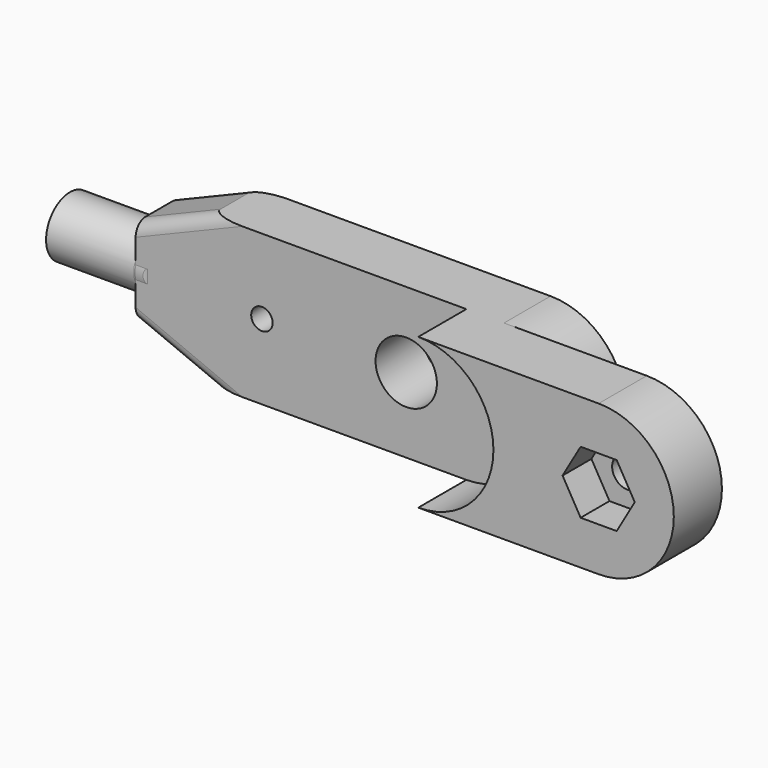
from build123d import *

# Parameters (mm, degrees)
F0_W         = 69.85
F0_H         = 15.875
F1_DEPTH     = 6.1468
F2_R         = 3.2385
F2_R_2       = 1.1303
F3_DEPTH     = 6.1478
F4_R         = 3.1496
F4_R_2       = 1.7272
F5_DEPTH     = 9.398
F7_T4_DEPTH  = 7.7320616198
F7_S5_R      = 3.1496
F7_T6_DEPTH  = 5
F7_T10_DEPTH = 7.7320616198
F7_S11_R     = 3.1496
F7_T12_DEPTH = 5
F9_DEPTH     = 25.4
F11_DEPTH    = 25.4
F13_DEPTH    = 6.35
F14_R        = 1.6256
F15_DEPTH    = 25.4
F17_DEPTH    = 3.81
F18_R        = 1.27


# Not quite as in the source:
# - a fillet or chamfer that OpenCascade refuses, or shapes differently, is made with other operations: its cross-section is extruded or revolved along the edge and cut away or added


with BuildPart() as f1:
    # F0 (on Front) → F1 (new body)
    with BuildSketch(Plane.XZ):
        Rectangle(F0_W, F0_H)
    extrude(amount=F1_DEPTH)

    # F2 (on face) → F3 (cut, through all)
    with BuildSketch(Plane.XZ.offset(6.1468)):
        with Locations((-6.35, 0)):
            Circle(F2_R)
        with Locations((-21.59, 0)):
            Circle(F2_R_2)
    extrude(amount=-F3_DEPTH, mode=Mode.SUBTRACT)

    # F4 (on face) → F5 (join)
    with BuildSketch(Plane(origin=(-34.925, 0, 0), x_dir=(0, -1, 0), z_dir=(-1, 0, 0))):
        with Locations((3.0734, 0)):
            Circle(F4_R)
        with Locations((3.0734, 0)):
            Circle(F4_R_2, mode=Mode.SUBTRACT)
    extrude(amount=F5_DEPTH)

    # F7: fillet of radius 1.27 on 6 edges, made by hand


with BuildPart() as f7_tool2:
    # F7_s3 → F7_t4 (new body)
    with BuildSketch(Plane.XY.offset(3.8660308099)):
        with BuildLine():
            ThreePointArc((-33.6540343146, -0.0004), (-34.5530256121, 0.3719743879), (-34.9254, 1.2709656854))
            Line((-34.9254, 1.2709656854), (-35.0525365685, 1.2709656854))
            ThreePointArc((-35.0525365685, 1.2709656854), (-35.0521365685, 0.6354828427), (-35.0521365685, 0))
            Line((-35.0521365685, 0), (-34.925, -0.1271365685))
            ThreePointArc((-34.925, -0.1271365685), (-34.2895171573, -0.1271365685), (-33.6540343146, -0.1275365685))
            Line((-33.6540343146, -0.1275365685), (-33.6540343146, -0.0004))
        make_face()
    extrude(amount=-F7_T4_DEPTH)

    # F7_s5 → F7_t6 (intersect, symmetric)
    with BuildSketch(Plane.YZ.offset(-34.4)):
        with Locations((-3.0734, 0)):
            Circle(F7_S5_R)
    extrude(amount=F7_T6_DEPTH, both=True, mode=Mode.INTERSECT)


with BuildPart() as f1_1:
    add(f1.part)

    # F7_t1: union F7_tool2
    add(f7_tool2.part)


with BuildPart() as f7_tool8:
    # F7_s9 → F7_t10 (new body)
    with BuildSketch(Plane.XY.offset(3.8660308099)):
        with BuildLine():
            ThreePointArc((-33.6540343146, -6.1464), (-34.5530256121, -6.5187743879), (-34.9254, -7.4177656854))
            Line((-34.9254, -7.4177656854), (-35.0525365685, -7.4177656854))
            ThreePointArc((-35.0525365685, -7.4177656854), (-35.0521365685, -6.7822828427), (-35.0521365685, -6.1468))
            Line((-35.0521365685, -6.1468), (-34.925, -6.0196634315))
            ThreePointArc((-34.925, -6.0196634315), (-34.2895171573, -6.0196634315), (-33.6540343146, -6.0192634315))
            Line((-33.6540343146, -6.0192634315), (-33.6540343146, -6.1464))
        make_face()
    extrude(amount=-F7_T10_DEPTH)

    # F7_s11 → F7_t12 (intersect, symmetric)
    with BuildSketch(Plane.YZ.offset(-34.4)):
        with Locations((-3.0734, 0)):
            Circle(F7_S11_R)
    extrude(amount=F7_T12_DEPTH, both=True, mode=Mode.INTERSECT)


with BuildPart() as f1_2:
    add(f1_1.part)

    # F7_t7: union F7_tool8
    add(f7_tool8.part)

    # F8 (on face) → F9 (cut)
    with BuildSketch(Plane.XZ.offset(6.1468)):
        Polygon((-34.925, 4.6355), (-26.9748, 7.9375), (-34.925, 7.9375), align=None)
        Polygon((-34.925, -7.9375), (-26.9748, -7.9375), (-34.925, -4.6355), align=None)
    extrude(amount=-F9_DEPTH, mode=Mode.SUBTRACT)

    # F10 (on face) → F11 (cut)
    with BuildSketch(Plane.XZ.offset(6.1468)):
        with BuildLine():
            ThreePointArc((3.9751, 7.9375), (11.9126, 0), (3.9751, -7.9375))
            Line((3.9751, -7.9375), (34.925, -7.9375))
            Line((34.925, -7.9375), (34.925, 7.9375))
            Line((34.925, 7.9375), (3.9751, 7.9375))
        make_face()
    extrude(amount=-F11_DEPTH, mode=Mode.SUBTRACT)

    # F12 (on face) → F13 (join)
    with BuildSketch(Plane.XZ.offset(6.1468)):
        with BuildLine():
            ThreePointArc((0, 7.9375), (7.9375, 0), (0, -7.9375))
            Line((0, -7.9375), (19.05, -7.9375))
            ThreePointArc((19.05, -7.9375), (26.9875, 0), (19.05, 7.9375))
            Line((19.05, 7.9375), (0, 7.9375))
        make_face()
    extrude(amount=F13_DEPTH)

    # F14 (on face) → F15 (cut)
    with BuildSketch(Plane.XZ.offset(12.4968)):
        with Locations((19.05, 0)):
            Circle(F14_R)
    extrude(amount=-F15_DEPTH, mode=Mode.SUBTRACT)

    # F16 (on face) → F17 (cut)
    with BuildSketch(Plane.XZ.offset(12.4968)):
        Polygon((22.8628211777, 0), (20.9564105889, 3.302), (17.1435894111, 3.302), (15.2371788223, 0), (17.1435894111, -3.302), (20.9564105889, -3.302), align=None)
    extrude(amount=-F17_DEPTH, mode=Mode.SUBTRACT)

    # F18
    f18_edges = [f1_2.edges().sort_by_distance(p)[0] for p in [
        (-30.9499, -6.1468, -6.2865),
        (-30.9499, 0, -6.2865),
        (-30.9499, 0, 6.2865),
        (-30.9499, -6.1468, 6.2865),
    ]]
    fillet(f18_edges, radius=F18_R)


solid = f1_2.part
